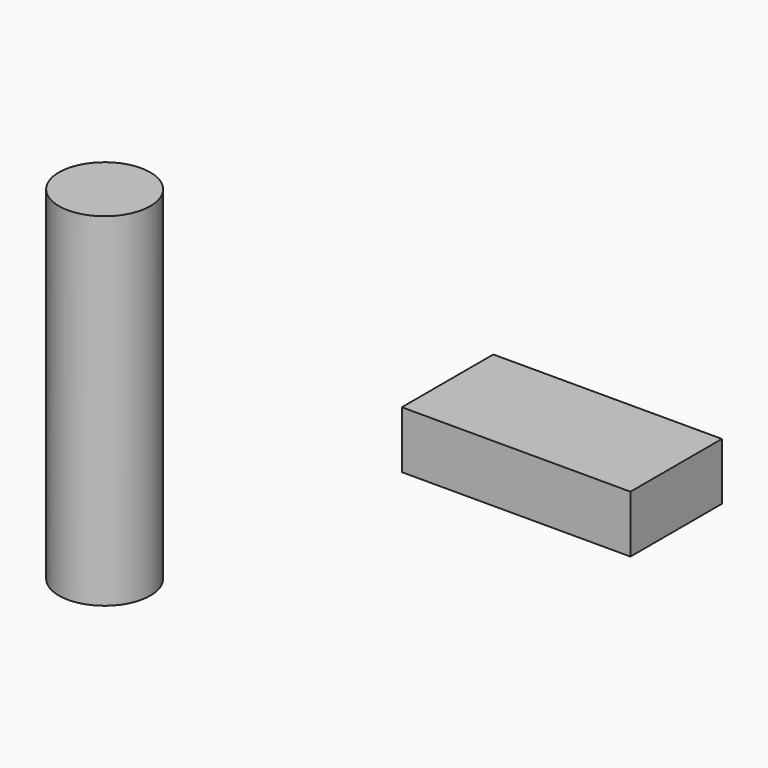
from build123d import *

# Parameters (mm, degrees)
F0_W          = 20
F0_H          = 10
F1_DEPTH      = 5
F0_R          = 4
F3_DEPTH      = 10
F3_DEPTH_BACK = 20


# Not quite as in the source:
# - a feature names something its author has since deleted; it is built from what else it names


with BuildPart() as f1:
    # F0 (on Top) → F1 (new body)
    with BuildSketch(Plane.XY):
        with Locations((40, 0)):
            Rectangle(F0_W, F0_H)
    extrude(amount=F1_DEPTH)


with BuildPart() as f3:
    # F0 (on Top) → F3 (new body, two sides)
    with BuildSketch(Plane.XY) as f3_sk:
        Circle(F0_R)
    extrude(amount=F3_DEPTH)
    extrude(f3_sk.sketch, amount=-F3_DEPTH_BACK)


solid = Compound([f1.part, f3.part])
